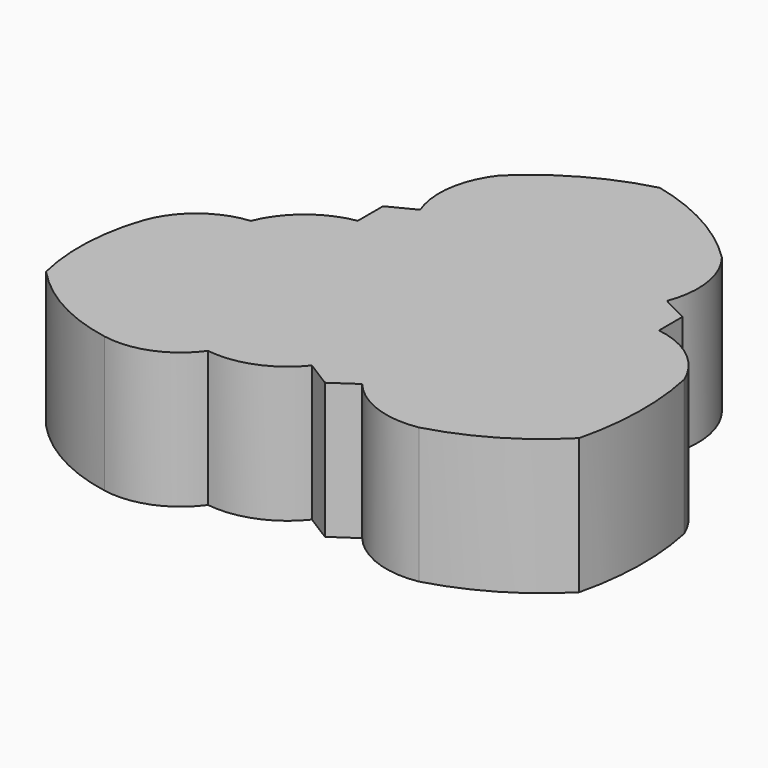
from build123d import *

# Parameters (mm, degrees)
F1_DEPTH = 11.1125


# Not quite as in the source:
# - a length typed as a fraction of an inch, garbled in the dataset ("3 / 203.2 mm" for 3/8 in), is restored


with BuildPart() as f1:
    # F0 (on Top) → F1 (new body)
    with BuildSketch(Plane.XY):
        with BuildLine():
            ThreePointArc((-0.1411418198, 20.1985444874), (-5.0054503986, 18.2564119782), (-9.2097157612, 15.1327075437))
            ThreePointArc((-9.2097157612, 15.1327075437), (-10.6205392688, 11.8246856933), (-10.2093555033, 8.2519613206))
            Line((-10.2093555033, 8.2519613206), (-12.369341217, 7.1464567445))
            Line((-12.369341217, 7.1464567445), (-12.369341217, 4.6386048198))
            Line((-12.369341217, 4.6386048198), (-12.369341217, 4.5682978211))
            ThreePointArc((-12.369341217, 4.5682978211), (-15.5930977879, 3.1185654947), (-17.7027139134, 0.2823972963))
            ThreePointArc((-17.7027139134, 0.2823972963), (-21.0452825194, -1.0603738309), (-23.1384971151, -3.9919692741))
            ThreePointArc((-23.1384971151, -3.9919692741), (-23.9954710425, -8.6613028545), (-23.5336683691, -13.3861117065))
            ThreePointArc((-23.5336683691, -13.3861117065), (-19.6562098094, -16.4130421994), (-15.0192606046, -18.054899429))
            ThreePointArc((-15.0192606046, -18.054899429), (-11.4338171794, -17.7079201351), (-8.5996589687, -15.484556372))
            ThreePointArc((-8.5996589687, -15.484556372), (-5.0294162563, -15.0523544446), (-2.1409380715, -12.9098966718))
            Line((-2.1409380715, -12.9098966718), (0, -14.2561570176))
            Line((0, -14.2561570176), (1.9696742658, -12.9098966718))
            ThreePointArc((1.9696742658, -12.9098966718), (4.9392756736, -15.0084468105), (8.560301624, -15.3410370587))
            ThreePointArc((8.560301624, -15.3410370587), (13.367982191, -13.3015402533), (17.4874793738, -10.0916987285))
            ThreePointArc((17.4874793738, -10.0916987285), (18.16772005, -4.8427956267), (17.6633565687, 0.4259166096))
            ThreePointArc((17.6633565687, 0.4259166096), (15.4847616458, 3.3168082822), (12.1560195839, 4.739132713))
            Line((12.1560195839, 4.739132713), (12.1560195839, 7.1464567445))
            Line((12.1560195839, 7.1464567445), (9.9960338703, 8.2519613206))
            ThreePointArc((9.9960338703, 8.2519613206), (10.4072176357, 11.8246856933), (8.9963941282, 15.1327075437))
            ThreePointArc((8.9963941282, 15.1327075437), (4.7823081966, 18.3053860292), (-0.1411418198, 20.1985444874))
        make_face()
    extrude(amount=F1_DEPTH)


solid = f1.part
